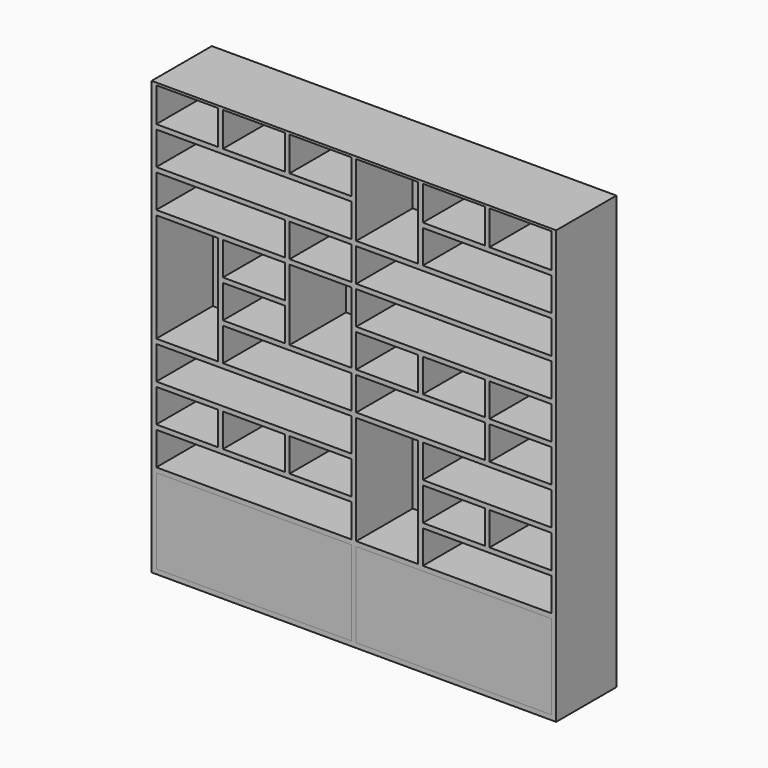
from build123d import *

# Parameters (mm, degrees)
F0_W     = 2150
F0_H     = 2300
F1_DEPTH = 400
F2_W     = 329.1666666667
F2_H     = 181.9444444444
F2_H_2   = 382.6388888889
F2_W_2   = 1037.5
F2_H_3   = 175.6944444444
F2_W_3   = 683.3333333333
F2_H_4   = 577.0833333333
F2_H_5   = 376.3888888889
F2_H_6   = 450
F3_DEPTH = 375
F4_DEPTH = 375
F5_T     = -15
F5_2_T   = -15


with BuildPart() as f1:
    # F0 (on Front) → F1 (new body)
    with BuildSketch(Plane.XZ):
        with Locations((0, 1150)):
            Rectangle(F0_W, F0_H)
    extrude(amount=F1_DEPTH)

    # F2 (on face) → F3 (cut, through all)
    with BuildSketch(Plane.XZ.offset(400)):
        with Locations((-885.4166666667, 2196.5277777778)):
            Rectangle(F2_W, F2_H)
        with Locations((-531.25, 2196.5277777778)):
            Rectangle(F2_W, F2_H)
        with Locations((-177.0833333333, 2196.5277777778)):
            Rectangle(F2_W, F2_H)
        with Locations((177.0833333333, 2096.1805555556)):
            Rectangle(F2_W, F2_H_2)
        with Locations((531.25, 2196.5277777778)):
            Rectangle(F2_W, F2_H)
        with Locations((885.4166666667, 2196.5277777778)):
            Rectangle(F2_W, F2_H)
        with Locations((-531.25, 1992.7083333333)):
            Rectangle(F2_W_2, F2_H_3)
        with Locations((708.3333333333, 1992.7083333333)):
            Rectangle(F2_W_3, F2_H_3)
        with Locations((-708.3333333333, 1792.0138888889)):
            Rectangle(F2_W_3, F2_H_3)
        with Locations((-177.0833333333, 1792.0138888889)):
            Rectangle(F2_W, F2_H_3)
        with Locations((531.25, 1792.0138888889)):
            Rectangle(F2_W_2, F2_H_3)
        with Locations((-885.4166666667, 1390.625)):
            Rectangle(F2_W, F2_H_4)
        with Locations((-531.25, 1591.3194444444)):
            Rectangle(F2_W, F2_H_3)
        with Locations((-531.25, 1390.625)):
            Rectangle(F2_W, F2_H_3)
        with Locations((-354.1666666667, 1189.9305555556)):
            Rectangle(F2_W_3, F2_H_3)
        with Locations((-177.0833333333, 1490.9722222222)):
            Rectangle(F2_W, F2_H_5)
        with Locations((531.25, 1591.3194444444)):
            Rectangle(F2_W_2, F2_H_3)
        with Locations((177.0833333333, 1390.625)):
            Rectangle(F2_W, F2_H_3)
        with Locations((531.25, 1390.625)):
            Rectangle(F2_W, F2_H_3)
        with Locations((885.4166666667, 1390.625)):
            Rectangle(F2_W, F2_H_3)
        with Locations((354.1666666667, 1189.9305555556)):
            Rectangle(F2_W_3, F2_H_3)
        with Locations((885.4166666667, 1189.9305555556)):
            Rectangle(F2_W, F2_H_3)
        with Locations((-531.25, 989.2361111111)):
            Rectangle(F2_W_2, F2_H_3)
        with Locations((-885.4166666667, 788.5416666667)):
            Rectangle(F2_W, F2_H_3)
        with Locations((-531.25, 788.5416666667)):
            Rectangle(F2_W, F2_H_3)
        with Locations((-177.0833333333, 788.5416666667)):
            Rectangle(F2_W, F2_H_3)
        with Locations((-531.25, 587.8472222222)):
            Rectangle(F2_W_2, F2_H_3)
        with Locations((177.0833333333, 788.5416666667)):
            Rectangle(F2_W, F2_H_4)
        with Locations((708.3333333333, 989.2361111111)):
            Rectangle(F2_W_3, F2_H_3)
        with Locations((531.25, 788.5416666667)):
            Rectangle(F2_W, F2_H_3)
        with Locations((885.4166666667, 788.5416666667)):
            Rectangle(F2_W, F2_H_3)
        with Locations((708.3333333333, 587.8472222222)):
            Rectangle(F2_W_3, F2_H_3)
        with Locations((-531.25, 250)):
            Rectangle(F2_W_2, F2_H_6)
        with Locations((531.25, 250)):
            Rectangle(F2_W_2, F2_H_6)
    extrude(amount=-F3_DEPTH, mode=Mode.SUBTRACT)


with BuildPart() as f4:
    # F2 (on face) → F4 (new body, through all)
    with BuildSketch(Plane.XZ.offset(400)):
        with Locations((-531.25, 250)):
            Rectangle(F2_W_2, F2_H_6)
    extrude(amount=-F4_DEPTH)

    # F5
    f5_openings = [f4.faces().sort_by_distance(p)[0] for p in [
        (-531.25, -212.5, 475),
    ]]
    offset(amount=F5_T, openings=f5_openings)


with BuildPart() as f4b:
    # F2 (on face) → F4, piece 2 (new body, through all)
    with BuildSketch(Plane.XZ.offset(400)):
        with Locations((531.25, 250)):
            Rectangle(F2_W_2, F2_H_6)
    extrude(amount=-F4_DEPTH)

    # F5#2
    f5_2_openings = [f4b.faces().sort_by_distance(p)[0] for p in [
        (531.25, -212.5, 475),
    ]]
    offset(amount=F5_2_T, openings=f5_2_openings)


solid = Compound([f1.part, f4.part, f4b.part])
